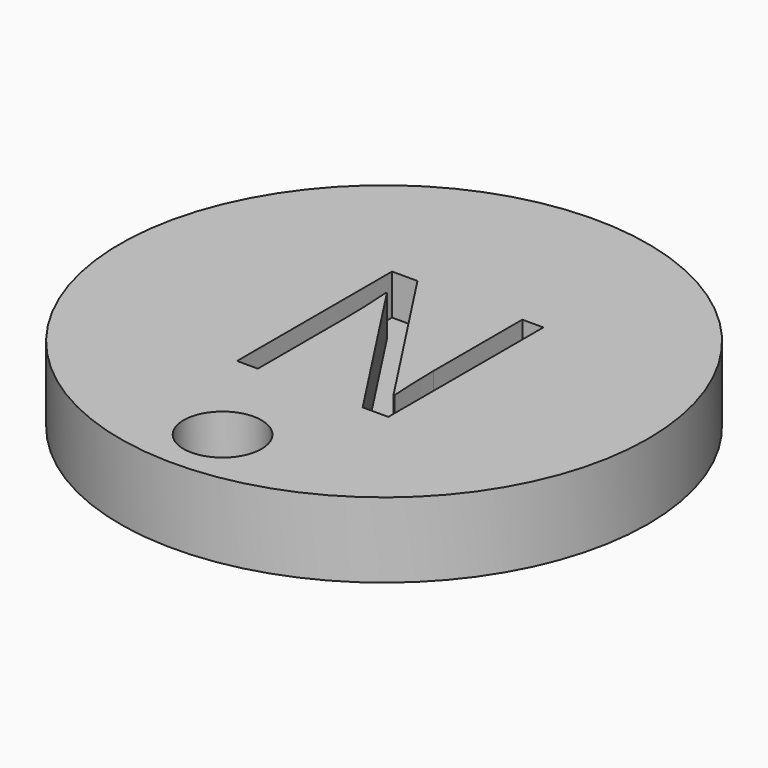
from build123d import *

# Parameters (mm, degrees)
F0_R         = 35.1556531311
F1_DEPTH     = 10
F2_R         = 5.1907195466
F3_DEPTH     = 66.4
F4_TEXT_SIZE = 36.1459614295
F5_DEPTH     = 5.4


# Not quite as in the source:
# - Text() gives the source's letters only with a copy of the font that has no kerning and outlines rounded to 1/6400 em; it was checked with that copy


with BuildPart() as f1:
    # F0 (on Top) → F1 (new body)
    with BuildSketch(Plane.XY):
        Circle(F0_R)
    extrude(amount=F1_DEPTH)

    # F2 (on Top) → F3 (cut)
    with BuildSketch(Plane.XY):
        with Locations((0, -26.8925968558)):
            Circle(F2_R)
    extrude(amount=F3_DEPTH, mode=Mode.SUBTRACT)

    # F4 (on face) → F5 (cut)
    with BuildSketch(Plane.XY.offset(10)):
        with Locations((-12.7233780804, -13.0125464129)):
            Text('N', F4_TEXT_SIZE, font='Open Sans', text_align=(TextAlign.LEFT, TextAlign.BOTTOM))
    extrude(amount=-F5_DEPTH, mode=Mode.SUBTRACT)


solid = f1.part
